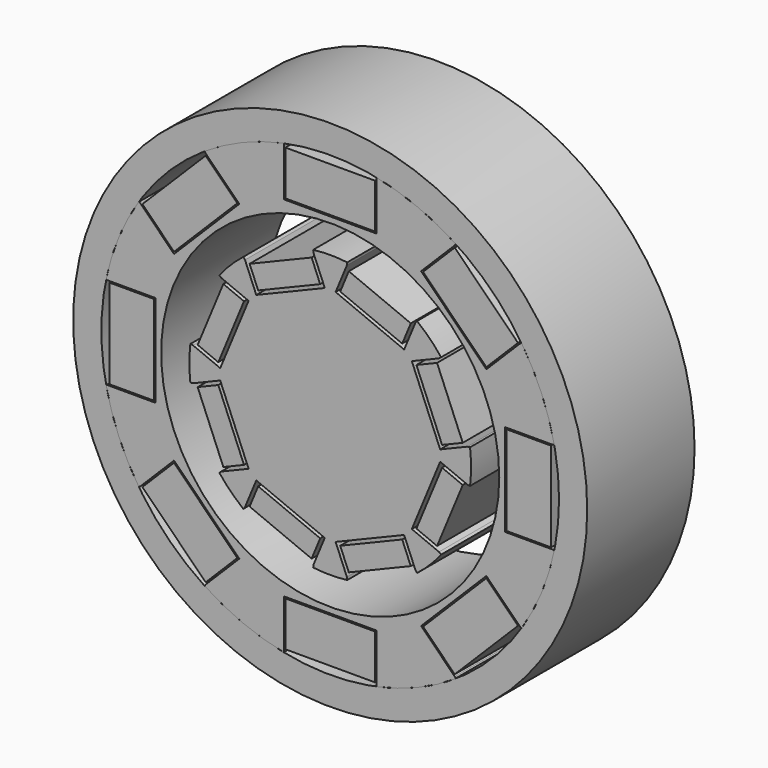
from build123d import *

# Parameters (mm, degrees)
F0_R     = 18.2433189176
F0_R_2   = 16.2433189176
F1_DEPTH = 9.525
F0_W     = 6.35
F0_H     = 3.175
F0_W_2   = 4.7625
F0_H_2   = 1.5875
F0_R_3   = 7.3592194389
F0_R_4   = 5.3592194389
F3_COUNT = 8
F5_DEPTH = 9.525
F6_R     = 12
F7_DEPTH = 9.525
F8_ANGLE = 22.5


# Not quite as in the source:
# - a length typed as a fraction of an inch, garbled in the dataset ("3 / 203.2 mm" for 3/8 in), is restored


with BuildPart() as f1:
    # F0 (on Front) → F1 (new body)
    with BuildSketch(Plane.XZ):
        Circle(F0_R)
        Circle(F0_R_2, mode=Mode.SUBTRACT)
    extrude(amount=F1_DEPTH)


with BuildPart() as f1b:
    # F0 (on Front) → F1, piece 2 (new body)
    with BuildSketch(Plane.XZ):
        with Locations((0, 14.0875)):
            Rectangle(F0_W, F0_H)
    extrude(amount=F1_DEPTH)


with BuildPart() as f1c:
    # F0 (on Front) → F1, piece 3 (new body)
    with BuildSketch(Plane.XZ):
        with Locations((0, 8.4029694389)):
            Rectangle(F0_W_2, F0_H_2)
    extrude(amount=F1_DEPTH)


with BuildPart() as f1d:
    # F0 (on Front) → F1, piece 4 (new body)
    with BuildSketch(Plane.XZ):
        Circle(F0_R_3)
        Circle(F0_R_4, mode=Mode.SUBTRACT)
    extrude(amount=F1_DEPTH)

    # F4 (on Front) → F5 (join)
    with BuildSketch(Plane.XZ):
        with BuildLine():
            ThreePointArc((5.2037539442, -5.2037539948), (6.799032208, -2.8162513709), (7.3592194389, 0))
            ThreePointArc((7.3592194389, 0), (6.7990322148, 2.8162513544), (5.2037539695, 5.2037539695))
            ThreePointArc((5.2037539695, 5.2037539695), (2.8162513544, 6.7990322148), (0, 7.3592194389))
            ThreePointArc((0, 7.3592194389), (-2.8162513413, 6.7990322203), (-5.2037539495, 5.2037539895))
            ThreePointArc((-5.2037539495, 5.2037539895), (-6.7990322094, 2.8162513675), (-7.3592194389, 0))
            ThreePointArc((-7.3592194389, 0), (-6.7990322148, -2.8162513544), (-5.2037539695, -5.2037539695))
            ThreePointArc((-5.2037539695, -5.2037539695), (-2.8162513544, -6.7990322148), (0, -7.3592194389))
            ThreePointArc((0, -7.3592194389), (2.8162513379, -6.7990322217), (5.2037539442, -5.2037539948))
        make_face()
        with BuildLine():
            Line((7.3592194389, -2.63125), (7.3592194389, 0))
            ThreePointArc((7.3592194389, 0), (6.799032208, -2.8162513709), (5.2037539442, -5.2037539948))
            Line((5.2037539442, -5.2037539948), (7.0643286875, -3.3431792515))
            Line((7.0643286875, -3.3431792515), (8.5404140932, -4.8192646572))
            Line((8.5404140932, -4.8192646572), (8.7090884873, -4.9144458202))
            ThreePointArc((8.7090884873, -4.9144458202), (9.2387953251, -3.8268343237), (9.6332934926, -2.6832175621))
            Line((9.6332934926, -2.6832175621), (9.4467194389, -2.63125))
            Line((9.4467194389, -2.63125), (7.3592194389, -2.63125))
        make_face()
        with BuildLine():
            ThreePointArc((5.2037539695, 5.2037539695), (6.7990322148, 2.8162513544), (7.3592194389, 0))
            Line((7.3592194389, 0), (7.3592194389, 2.63125))
            Line((7.3592194389, 2.63125), (9.4467194389, 2.63125))
            Line((9.4467194389, 2.63125), (9.6332934926, 2.6832175621))
            ThreePointArc((9.6332934926, 2.6832175621), (9.2387953251, 3.8268343237), (8.7090884873, 4.9144458202))
            Line((8.7090884873, 4.9144458202), (8.5404140932, 4.8192646572))
            Line((8.5404140932, 4.8192646572), (7.0643286875, 3.3431792515))
            Line((7.0643286875, 3.3431792515), (5.2037539695, 5.2037539695))
        make_face()
        with BuildLine():
            ThreePointArc((0, 7.3592194389), (2.8162513544, 6.7990322148), (5.2037539695, 5.2037539695))
            Line((5.2037539695, 5.2037539695), (3.3431792515, 7.0643286875))
            Line((3.3431792515, 7.0643286875), (4.8192646572, 8.5404140932))
            Line((4.8192646572, 8.5404140932), (4.9144458202, 8.7090884873))
            ThreePointArc((4.9144458202, 8.7090884873), (3.8268343237, 9.2387953251), (2.6832175621, 9.6332934926))
            Line((2.6832175621, 9.6332934926), (2.63125, 9.4467194389))
            Line((2.63125, 9.4467194389), (2.63125, 7.3592194389))
            Line((2.63125, 7.3592194389), (0, 7.3592194389))
        make_face()
        with BuildLine():
            Line((3.3431792515, -7.0643286875), (5.2037539442, -5.2037539948))
            ThreePointArc((5.2037539442, -5.2037539948), (2.8162513379, -6.7990322217), (0, -7.3592194389))
            Line((0, -7.3592194389), (2.63125, -7.3592194389))
            Line((2.63125, -7.3592194389), (2.63125, -9.4467194389))
            Line((2.63125, -9.4467194389), (2.6832175621, -9.6332934926))
            ThreePointArc((2.6832175621, -9.6332934926), (3.8268343237, -9.2387953251), (4.9144458202, -8.7090884873))
            Line((4.9144458202, -8.7090884873), (4.8192646572, -8.5404140932))
            Line((4.8192646572, -8.5404140932), (3.3431792515, -7.0643286875))
        make_face()
        with BuildLine():
            ThreePointArc((-5.2037539495, 5.2037539895), (-2.8162513413, 6.7990322203), (0, 7.3592194389))
            Line((0, 7.3592194389), (-2.63125, 7.3592194389))
            Line((-2.63125, 7.3592194389), (-2.63125, 9.4467194389))
            Line((-2.63125, 9.4467194389), (-2.6832175621, 9.6332934926))
            ThreePointArc((-2.6832175621, 9.6332934926), (-3.8268343237, 9.2387953251), (-4.9144458202, 8.7090884873))
            Line((-4.9144458202, 8.7090884873), (-4.8192646572, 8.5404140932))
            Line((-4.8192646572, 8.5404140932), (-3.3431792515, 7.0643286875))
            Line((-3.3431792515, 7.0643286875), (-5.2037539495, 5.2037539895))
        make_face()
        with BuildLine():
            Line((-2.63125, -7.3592194389), (0, -7.3592194389))
            ThreePointArc((0, -7.3592194389), (-2.8162513544, -6.7990322148), (-5.2037539695, -5.2037539695))
            Line((-5.2037539695, -5.2037539695), (-3.3431792515, -7.0643286875))
            Line((-3.3431792515, -7.0643286875), (-4.8192646572, -8.5404140932))
            Line((-4.8192646572, -8.5404140932), (-4.9144458202, -8.7090884873))
            ThreePointArc((-4.9144458202, -8.7090884873), (-3.8268343237, -9.2387953251), (-2.6832175621, -9.6332934926))
            Line((-2.6832175621, -9.6332934926), (-2.63125, -9.4467194389))
            Line((-2.63125, -9.4467194389), (-2.63125, -7.3592194389))
        make_face()
        with BuildLine():
            ThreePointArc((-7.3592194389, 0), (-6.7990322094, 2.8162513675), (-5.2037539495, 5.2037539895))
            Line((-5.2037539495, 5.2037539895), (-7.0643286875, 3.3431792515))
            Line((-7.0643286875, 3.3431792515), (-8.5404140932, 4.8192646572))
            Line((-8.5404140932, 4.8192646572), (-8.7090884873, 4.9144458202))
            ThreePointArc((-8.7090884873, 4.9144458202), (-9.2387953251, 3.8268343237), (-9.6332934926, 2.6832175621))
            Line((-9.6332934926, 2.6832175621), (-9.4467194389, 2.63125))
            Line((-9.4467194389, 2.63125), (-7.3592194389, 2.63125))
            Line((-7.3592194389, 2.63125), (-7.3592194389, 0))
        make_face()
        with BuildLine():
            Line((-7.0643286875, -3.3431792515), (-5.2037539695, -5.2037539695))
            ThreePointArc((-5.2037539695, -5.2037539695), (-6.7990322148, -2.8162513544), (-7.3592194389, 0))
            Line((-7.3592194389, 0), (-7.3592194389, -2.63125))
            Line((-7.3592194389, -2.63125), (-9.4467194389, -2.63125))
            Line((-9.4467194389, -2.63125), (-9.6332934926, -2.6832175621))
            ThreePointArc((-9.6332934926, -2.6832175621), (-9.2387953251, -3.8268343237), (-8.7090884873, -4.9144458202))
            Line((-8.7090884873, -4.9144458202), (-8.5404140932, -4.8192646572))
            Line((-8.5404140932, -4.8192646572), (-7.0643286875, -3.3431792515))
        make_face()
    extrude(amount=F5_DEPTH)


with BuildPart() as f3_1:
    # F3: instance of F1c
    add(f1c.part.rotate(Axis((0, 60.4257024825, 0), (0, 1, 0)), 1 * 360 / F3_COUNT))


with BuildPart() as f3_2:
    # F3: instance of F1c
    add(f1c.part.rotate(Axis((0, 60.4257024825, 0), (0, 1, 0)), 2 * 360 / F3_COUNT))


with BuildPart() as f3_3:
    # F3: instance of F1c
    add(f1c.part.rotate(Axis((0, 60.4257024825, 0), (0, 1, 0)), 3 * 360 / F3_COUNT))


with BuildPart() as f3_4:
    # F3: instance of F1c
    add(f1c.part.rotate(Axis((0, 60.4257024825, 0), (0, 1, 0)), 4 * 360 / F3_COUNT))


with BuildPart() as f3_5:
    # F3: instance of F1c
    add(f1c.part.rotate(Axis((0, 60.4257024825, 0), (0, 1, 0)), 5 * 360 / F3_COUNT))


with BuildPart() as f3_6:
    # F3: instance of F1c
    add(f1c.part.rotate(Axis((0, 60.4257024825, 0), (0, 1, 0)), 6 * 360 / F3_COUNT))


with BuildPart() as f3_7:
    # F3: instance of F1c
    add(f1c.part.rotate(Axis((0, 60.4257024825, 0), (0, 1, 0)), 7 * 360 / F3_COUNT))


with BuildPart() as f3_8:
    # F3: instance of F1b
    add(f1b.part.rotate(Axis((0, 60.4257024825, 0), (0, 1, 0)), 1 * 360 / F3_COUNT))


with BuildPart() as f3_9:
    # F3: instance of F1b
    add(f1b.part.rotate(Axis((0, 60.4257024825, 0), (0, 1, 0)), 2 * 360 / F3_COUNT))


with BuildPart() as f3_10:
    # F3: instance of F1b
    add(f1b.part.rotate(Axis((0, 60.4257024825, 0), (0, 1, 0)), 3 * 360 / F3_COUNT))


with BuildPart() as f3_11:
    # F3: instance of F1b
    add(f1b.part.rotate(Axis((0, 60.4257024825, 0), (0, 1, 0)), 4 * 360 / F3_COUNT))


with BuildPart() as f3_12:
    # F3: instance of F1b
    add(f1b.part.rotate(Axis((0, 60.4257024825, 0), (0, 1, 0)), 5 * 360 / F3_COUNT))


with BuildPart() as f3_13:
    # F3: instance of F1b
    add(f1b.part.rotate(Axis((0, 60.4257024825, 0), (0, 1, 0)), 6 * 360 / F3_COUNT))


with BuildPart() as f3_14:
    # F3: instance of F1b
    add(f1b.part.rotate(Axis((0, 60.4257024825, 0), (0, 1, 0)), 7 * 360 / F3_COUNT))


with BuildPart() as f7:
    # F6 (on Front) → F7 (new body)
    with BuildSketch(Plane.XZ):
        with BuildLine():
            Line((-13.4703841816, 8.8388347648), (-13.5807037745, 8.9112229491))
            ThreePointArc((-13.5807037745, 8.9112229491), (-15.006869888, 6.2160490364), (-15.9041939082, 3.3018215562))
            Line((-15.9041939082, 3.3018215562), (-15.775, 3.275))
            Line((-15.775, 3.275), (-12.4, 3.275))
            Line((-12.4, 3.275), (-12.4, -3.275))
            Line((-12.4, -3.275), (-15.775, -3.275))
            Line((-15.775, -3.275), (-15.9041939082, -3.3018215562))
            ThreePointArc((-15.9041939082, -3.3018215562), (-15.006869888, -6.2160490364), (-13.5807037745, -8.9112229491))
            Line((-13.5807037745, -8.9112229491), (-13.4703841816, -8.8388347648))
            Line((-13.4703841816, -8.8388347648), (-11.0838987951, -6.4523493783))
            Line((-11.0838987951, -6.4523493783), (-6.4523493783, -11.0838987951))
            Line((-6.4523493783, -11.0838987951), (-8.8388347648, -13.4703841816))
            Line((-8.8388347648, -13.4703841816), (-8.9112229491, -13.5807037745))
            ThreePointArc((-8.9112229491, -13.5807037745), (-6.2160490364, -15.006869888), (-3.3018215562, -15.9041939082))
            Line((-3.3018215562, -15.9041939082), (-3.275, -15.775))
            Line((-3.275, -15.775), (-3.275, -12.4))
            Line((-3.275, -12.4), (3.275, -12.4))
            Line((3.275, -12.4), (3.275, -15.775))
            Line((3.275, -15.775), (3.3018215562, -15.9041939082))
            ThreePointArc((3.3018215562, -15.9041939082), (6.2160490364, -15.006869888), (8.9112229491, -13.5807037745))
            Line((8.9112229491, -13.5807037745), (8.8388347648, -13.4703841816))
            Line((8.8388347648, -13.4703841816), (6.4523493783, -11.0838987951))
            Line((6.4523493783, -11.0838987951), (11.0838987951, -6.4523493783))
            Line((11.0838987951, -6.4523493783), (13.4703841816, -8.8388347648))
            Line((13.4703841816, -8.8388347648), (13.5807037745, -8.9112229491))
            ThreePointArc((13.5807037745, -8.9112229491), (15.006869888, -6.2160490364), (15.9041939082, -3.3018215562))
            Line((15.9041939082, -3.3018215562), (15.775, -3.275))
            Line((15.775, -3.275), (12.4, -3.275))
            Line((12.4, -3.275), (12.4, 3.275))
            Line((12.4, 3.275), (15.775, 3.275))
            Line((15.775, 3.275), (15.9041939082, 3.3018215562))
            ThreePointArc((15.9041939082, 3.3018215562), (15.006869888, 6.2160490364), (13.5807037745, 8.9112229491))
            Line((13.5807037745, 8.9112229491), (13.4703841816, 8.8388347648))
            Line((13.4703841816, 8.8388347648), (11.0838987951, 6.4523493783))
            Line((11.0838987951, 6.4523493783), (6.4523493783, 11.0838987951))
            Line((6.4523493783, 11.0838987951), (8.8388347648, 13.4703841816))
            Line((8.8388347648, 13.4703841816), (8.9112229491, 13.5807037745))
            ThreePointArc((8.9112229491, 13.5807037745), (6.2160490364, 15.006869888), (3.3018215562, 15.9041939082))
            Line((3.3018215562, 15.9041939082), (3.275, 15.775))
            Line((3.275, 15.775), (3.275, 12.4))
            Line((3.275, 12.4), (-3.275, 12.4))
            Line((-3.275, 12.4), (-3.275, 15.775))
            Line((-3.275, 15.775), (-3.3018215562, 15.9041939082))
            ThreePointArc((-3.3018215562, 15.9041939082), (-6.2160490364, 15.006869888), (-8.9112229491, 13.5807037745))
            Line((-8.9112229491, 13.5807037745), (-8.8388347648, 13.4703841816))
            Line((-8.8388347648, 13.4703841816), (-6.4523493783, 11.0838987951))
            Line((-6.4523493783, 11.0838987951), (-11.0838987951, 6.4523493783))
            Line((-11.0838987951, 6.4523493783), (-13.4703841816, 8.8388347648))
        make_face()
        Circle(F6_R, mode=Mode.SUBTRACT)
    extrude(amount=F7_DEPTH)


with BuildPart() as f3_7_1:
    # F8: moved
    add(f3_7.part.rotate(Axis((0, 60.4257024825, 0), (0, 1, 0)), F8_ANGLE))


with BuildPart() as f1c_1:
    # F8: moved
    add(f1c.part.rotate(Axis((0, 60.4257024825, 0), (0, 1, 0)), F8_ANGLE))


with BuildPart() as f3_1_1:
    # F8: moved
    add(f3_1.part.rotate(Axis((0, 60.4257024825, 0), (0, 1, 0)), F8_ANGLE))


with BuildPart() as f3_2_1:
    # F8: moved
    add(f3_2.part.rotate(Axis((0, 60.4257024825, 0), (0, 1, 0)), F8_ANGLE))


with BuildPart() as f3_3_1:
    # F8: moved
    add(f3_3.part.rotate(Axis((0, 60.4257024825, 0), (0, 1, 0)), F8_ANGLE))


with BuildPart() as f3_4_1:
    # F8: moved
    add(f3_4.part.rotate(Axis((0, 60.4257024825, 0), (0, 1, 0)), F8_ANGLE))


with BuildPart() as f3_5_1:
    # F8: moved
    add(f3_5.part.rotate(Axis((0, 60.4257024825, 0), (0, 1, 0)), F8_ANGLE))


with BuildPart() as f3_6_1:
    # F8: moved
    add(f3_6.part.rotate(Axis((0, 60.4257024825, 0), (0, 1, 0)), F8_ANGLE))


with BuildPart() as f1d_1:
    # F8: moved
    add(f1d.part.rotate(Axis((0, 60.4257024825, 0), (0, 1, 0)), F8_ANGLE))


solid = Compound([f1.part, f1b.part, f3_8.part, f3_9.part, f3_10.part, f3_11.part, f3_12.part, f3_13.part, f3_14.part, f7.part, f3_7_1.part, f1c_1.part, f3_1_1.part, f3_2_1.part, f3_3_1.part, f3_4_1.part, f3_5_1.part, f3_6_1.part, f1d_1.part])
